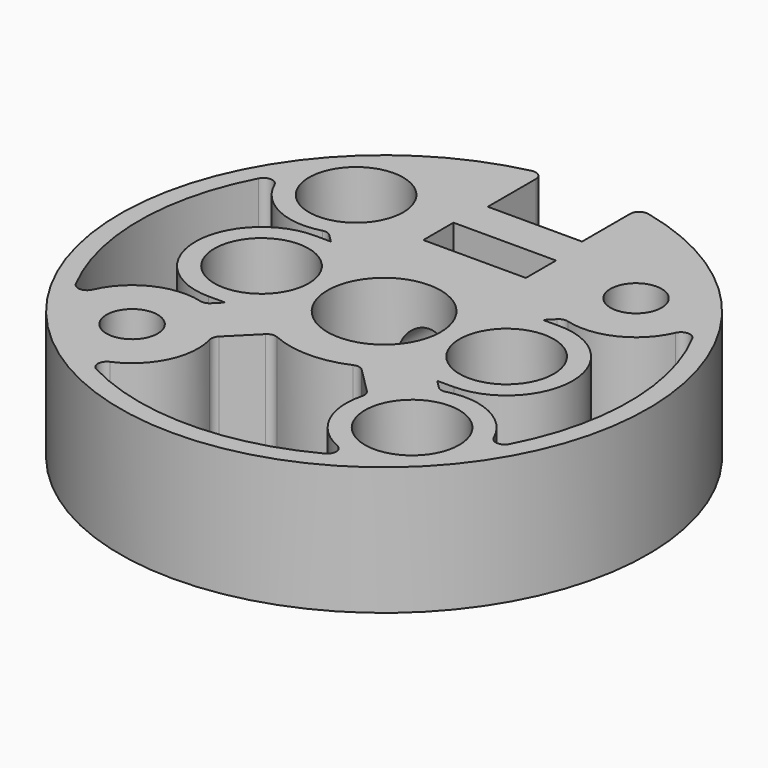
from build123d import *

# Parameters (mm, degrees)
F0_R      = 2.15265
F1_DEPTH  = 10.795
F2_R      = 2.15265
F3_REACH  = 44.1896136501
F6_R      = 3.96875
F7_DEPTH  = 6.35
F8_R      = 3.96875
F9_DEPTH  = 7.62
F11_DEPTH = 10.795
F12_R     = 2.15265
F13_REACH = 44.1896136501
F14_R     = 0.762
F18_DEPTH = 3.175
F19_R     = 3.96875
F19_R_2   = 2.15265
F21_DEPTH = 6.0325
F23_DEPTH = 10.795
F24_R     = 0.762


# Not quite as in the source:
# - a feature of the source that left no trace in its solid (it failed there, or was rolled back) is left out
# - a pattern or mirror of a feature is missing from the dataset's text; its kind, count and spacing are read off the source's solid


with BuildPart() as f1:
    # F0 (on Top) → F1 (new body)
    with BuildSketch(Plane.XY):
        with BuildLine():
            Line((3.96875, 15.875), (0, 15.875))
            Line((0, 15.875), (-3.96875, 15.875))
            Line((-3.96875, 15.875), (-3.96875, 21.8677764859))
            ThreePointArc((-3.96875, 21.8677764859), (0, -22.225), (3.96875, 21.8677764859))
            Line((3.96875, 21.8677764859), (3.96875, 15.875))
        make_face()
        with Locations((-11.7865861589, -11.7865861589)):
            Circle(F0_R, mode=Mode.SUBTRACT)
        with Locations((11.7865861589, -11.7865861589)):
            Circle(F0_R, mode=Mode.SUBTRACT)
        with Locations((-10.31875, 0)):
            Circle(F0_R, mode=Mode.SUBTRACT)
        with Locations((-11.7865861589, 11.7865861589)):
            Circle(F0_R, mode=Mode.SUBTRACT)
        with BuildLine():
            ThreePointArc((4.7625, 0), (-3.3675960454, -3.3675960454), (0, 4.7625))
            ThreePointArc((0, 4.7625), (3.3675960454, 3.3675960454), (4.7625, 0))
        make_face(mode=Mode.SUBTRACT)
        with Locations((10.31875, 0)):
            Circle(F0_R, mode=Mode.SUBTRACT)
        with Locations((11.7865861589, 11.7865861589)):
            Circle(F0_R, mode=Mode.SUBTRACT)
    extrude(amount=F1_DEPTH)

    f3_end = f1.faces().sort_by_distance((0, -4.7625, 5.3975))[0]
    # F2 (on face) → F3 (cut, up to a face of the model that its end follows)
    with BuildSketch(Plane(origin=(0, 15.875, 0), x_dir=(-1, 0, 0), z_dir=(0, 1, 0))):
        with Locations((0, 5.3975)):
            Circle(F2_R)
    f3_long = extrude(amount=-F3_REACH, mode=Mode.PRIVATE)
    add(split(f3_long, bisect_by=f3_end, keep=Keep.ALL, mode=Mode.PRIVATE).solids().sort_by_distance((0, 15.875, 5.3975))[0], mode=Mode.SUBTRACT)

    # F6 (on face) → F7 (cut, through all)
    with BuildSketch(Plane.XY.offset(10.795)):
        with Locations((-11.7865861589, 11.7865861589)):
            Circle(F6_R)
        with Locations((11.7865861589, -11.7865861589)):
            Circle(F6_R)
    extrude(amount=-F7_DEPTH, mode=Mode.SUBTRACT)

    # F8 (on face) → F9 (cut, through all)
    with BuildSketch(Plane(origin=(0, 0, 0), x_dir=(1, 0, 0), z_dir=(0, 0, -1))):
        with Locations((11.7865861589, -11.7865861589)):
            Circle(F8_R)
        with Locations((-11.7865861589, 11.7865861589)):
            Circle(F8_R)
    extrude(amount=-F9_DEPTH, mode=Mode.SUBTRACT)

    # F10 (on face) → F11 (cut, through all)
    with BuildSketch(Plane.XY.offset(10.795)):
        with BuildLine():
            ThreePointArc((-9.9206262673, 6.5530302219), (-14.7565267097, 7.0906978311), (-17.3148424047, 11.229543123))
            ThreePointArc((-17.3148424047, 11.229543123), (-20.6375, 0), (-17.3148424047, -11.229543123))
            ThreePointArc((-17.3148424047, -11.229543123), (-14.7565267097, -7.0906978311), (-9.9206262673, -6.5530302219))
            Line((-9.9206262673, -6.5530302219), (-8.9238460454, -5.55625))
            Line((-8.9238460454, -5.55625), (-10.31875, -5.55625))
            ThreePointArc((-10.31875, -5.55625), (-15.875, 0), (-10.31875, 5.55625))
            Line((-10.31875, 5.55625), (-8.9238460454, 5.55625))
            Line((-8.9238460454, 5.55625), (-9.9206262673, 6.5530302219))
        make_face()
    f11 = extrude(amount=-F11_DEPTH, mode=Mode.SUBTRACT)

    # F11_copies: F11 across plane
    add(f11.mirror(Plane(origin=(0, 0, 0), x_dir=(0, 0, 1), z_dir=(1, 0, 0))), mode=Mode.SUBTRACT)

    f13_end = f1.faces().sort_by_distance((0, -4.7625, 5.3975))[0]
    # F12 (on face) → F13 (cut, up to a face of the model that its end follows)
    with BuildSketch(Plane(origin=(0, 15.875, 0), x_dir=(-1, 0, 0), z_dir=(0, 1, 0))):
        with Locations((0, 5.3975)):
            Circle(F12_R)
    f13_long = extrude(amount=-F13_REACH, mode=Mode.PRIVATE)
    add(split(f13_long, bisect_by=f13_end, keep=Keep.TOP, mode=Mode.PRIVATE), mode=Mode.SUBTRACT)

    # F14
    f14_edges = [f1.edges().sort_by_distance(p)[0] for p in [
        (-17.314842, -11.229543, 5.3975),
        (-17.314842, 11.229543, 5.3975),
        (3.96875, 21.867776, 5.3975),
        (-3.96875, 21.867776, 5.3975),
        (-9.920626, 6.55303, 5.3975),
        (-9.920626, -6.55303, 5.3975),
        (9.920626, 6.55303, 5.3975),
        (9.920626, -6.55303, 5.3975),
        (17.314842, -11.229543, 5.3975),
        (17.314842, 11.229543, 5.3975),
    ]]
    fillet(f14_edges, radius=F14_R)

    # F17 (on offset) → F18 (cut)
    with BuildSketch(Plane(origin=(0, 12.7, 0), x_dir=(-1, 0, 0), z_dir=(0, 1, 0))):
        Polygon((-4.318, 7.8904984624), (-4.318, 2.9045015376), (-2.0368864232, 1.5875), (0, 0.4115030753), (2.0368864232, 1.5875), (4.318, 2.9045015376), (4.318, 7.8904984624), (4.318, 10.795), (-4.318, 10.795), align=None)
        Polygon((0, 0.4115030753), (-2.0368864232, 1.5875), (-2.0368864232, 0), (2.0368864232, 0), (2.0368864232, 1.5875), align=None)
    extrude(amount=-F18_DEPTH, mode=Mode.SUBTRACT)

    # F19 (on face) → F21 (cut, through all)
    with BuildSketch(Plane.XY.offset(10.795)):
        with Locations((-10.31875, 0)):
            Circle(F19_R)
        with Locations((-10.31875, 0)):
            Circle(F19_R_2, mode=Mode.SUBTRACT)
        with Locations((10.31875, 0)):
            Circle(F19_R)
        with Locations((10.31875, 0)):
            Circle(F19_R_2, mode=Mode.SUBTRACT)
    extrude(amount=-F21_DEPTH, mode=Mode.SUBTRACT)

    # F22 (on face) → F23 (cut, through all)
    with BuildSketch(Plane.XY.offset(10.795)):
        with BuildLine():
            Line((-3.6703384477, -7.0379344931), (-6.5530302219, -9.9206262673))
            ThreePointArc((-6.5530302219, -9.9206262673), (-7.0906978311, -14.7565267097), (-11.229543123, -17.3148424047))
            ThreePointArc((-11.229543123, -17.3148424047), (0, -20.6375), (11.229543123, -17.3148424047))
            ThreePointArc((11.229543123, -17.3148424047), (7.0906978311, -14.7565267097), (6.5530302219, -9.9206262673))
            Line((6.5530302219, -9.9206262673), (3.6703384477, -7.0379344931))
            ThreePointArc((3.6703384477, -7.0379344931), (0, -7.9375), (-3.6703384477, -7.0379344931))
        make_face()
    extrude(amount=-F23_DEPTH, mode=Mode.SUBTRACT)

    # F24
    f24_edges = [f1.edges().sort_by_distance(p)[0] for p in [
        (3.670338, -7.037934, 5.3975),
        (6.55303, -9.920626, 5.3975),
        (11.229543, -17.314842, 5.3975),
        (-11.229543, -17.314842, 5.3975),
        (-6.55303, -9.920626, 5.3975),
        (-3.670338, -7.037934, 5.3975),
    ]]
    fillet(f24_edges, radius=F24_R)


solid = f1.part
